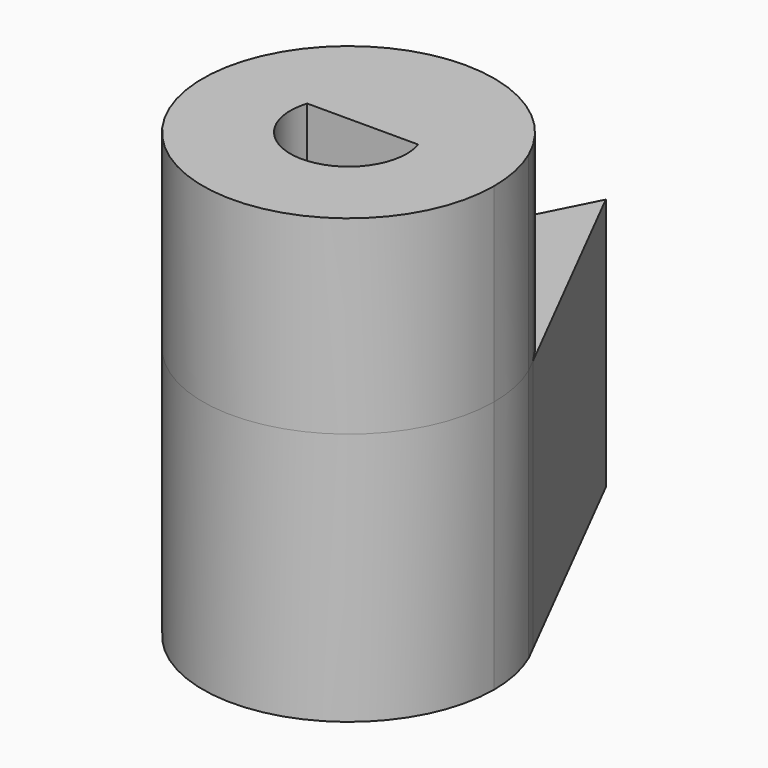
from build123d import *

# Parameters (mm, degrees)
F1_DEPTH = 9.525
F2_DEPTH = 12.7


with BuildPart() as f1:
    # F0 (on Top) → F1 (new body)
    with BuildSketch(Plane.XY):
        with BuildLine():
            ThreePointArc((-6.7061053414, 2.890442423), (-1.4756645952, -7.1518473315), (7.3025, 0))
            ThreePointArc((7.3025, 0), (7.1473488528, 1.4973011139), (6.6884881888, 2.9309779936))
            Line((6.6884881888, 2.9309779936), (6.3166219962, 3.6642588347))
            ThreePointArc((6.3166219962, 3.6642588347), (0.0208084361, 7.3024703532), (-6.2956369305, 3.7001975474))
            Line((-6.2956369305, 3.7001975474), (-6.7061053414, 2.890442423))
        make_face()
        with BuildLine():
            ThreePointArc((2.7824305921, 0.889), (2.8861497501, 0.4498673362), (2.921, 0))
            ThreePointArc((2.921, 0), (-0.4498673362, -2.8861497501), (-2.7824305921, 0.889))
            ThreePointArc((-2.7824305921, 0.889), (0, 2.921), (2.7824305921, 0.889))
        make_face(mode=Mode.SUBTRACT)
        with BuildLine():
            Line((-2.7824305921, 0.889), (2.7824305921, 0.889))
            ThreePointArc((2.7824305921, 0.889), (0, 2.921), (-2.7824305921, 0.889))
        make_face()
    extrude(amount=F1_DEPTH)


with BuildPart() as f2:
    # F0 (on Top) → F2 (new body)
    with BuildSketch(Plane.XY):
        with BuildLine():
            ThreePointArc((-6.7061053414, 2.890442423), (-1.4756645952, -7.1518473315), (7.3025, 0))
            ThreePointArc((7.3025, 0), (7.1473488528, 1.4973011139), (6.6884881888, 2.9309779936))
            Line((6.6884881888, 2.9309779936), (6.3166219962, 3.6642588347))
            ThreePointArc((6.3166219962, 3.6642588347), (0.0208084361, 7.3024703532), (-6.2956369305, 3.7001975474))
            Line((-6.2956369305, 3.7001975474), (-6.7061053414, 2.890442423))
        make_face()
        with BuildLine():
            ThreePointArc((2.7824305921, 0.889), (2.8861497501, 0.4498673362), (2.921, 0))
            ThreePointArc((2.921, 0), (-0.4498673362, -2.8861497501), (-2.7824305921, 0.889))
            ThreePointArc((-2.7824305921, 0.889), (0, 2.921), (2.7824305921, 0.889))
        make_face(mode=Mode.SUBTRACT)
        with BuildLine():
            ThreePointArc((-6.2956369305, 3.7001975474), (0.0208084361, 7.3024703532), (6.3166219962, 3.6642588347))
            Line((6.3166219962, 3.6642588347), (0, 16.1199700087))
            Line((0, 16.1199700087), (-6.2956369305, 3.7001975474))
        make_face()
        with BuildLine():
            ThreePointArc((-2.7824305921, 0.889), (-0.4498673362, -2.8861497501), (2.921, 0))
            ThreePointArc((2.921, 0), (2.8861497501, 0.4498673362), (2.7824305921, 0.889))
            Line((2.7824305921, 0.889), (-2.7824305921, 0.889))
        make_face()
        with BuildLine():
            Line((-2.7824305921, 0.889), (2.7824305921, 0.889))
            ThreePointArc((2.7824305921, 0.889), (0, 2.921), (-2.7824305921, 0.889))
        make_face()
    extrude(amount=-F2_DEPTH)


solid = Compound([f1.part, f2.part])
